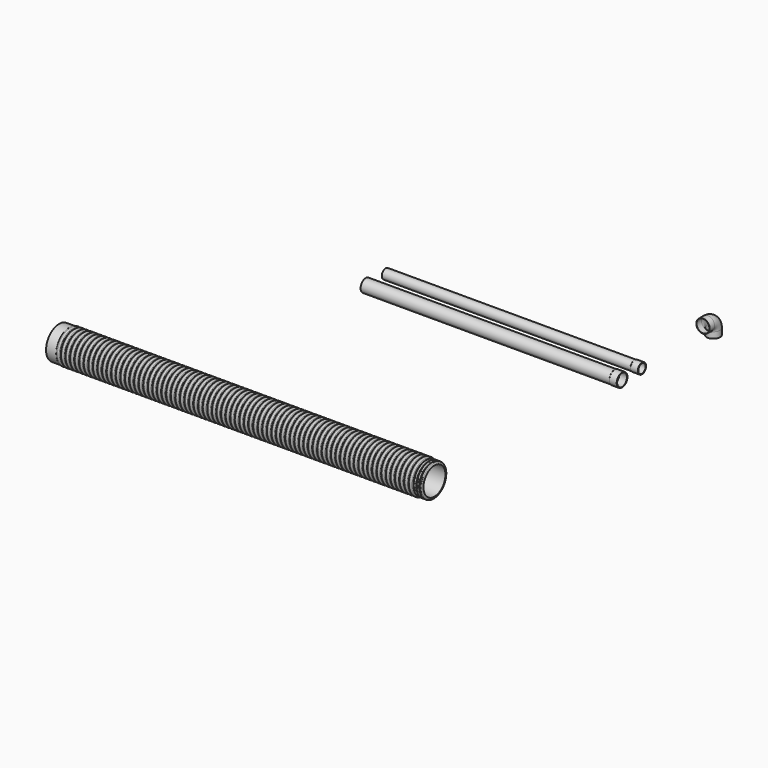
from build123d import *

# Parameters (mm, degrees)
F0_R      = 81.28
F0_R_2    = 76.2
F1_DEPTH  = 4140.2
F0_R_3    = 106.68
F0_R_4    = 101.6
F0_R_5    = 111.76
F2_DEPTH  = 127
F0_R_6    = 86.36
F3_DEPTH  = 127
F4_SIZE   = 5.07999
F4_2_SIZE = 5.07999
F9_R      = 111.76
F9_R_2    = 106.68


# Not quite as in the source:
# - a fillet or chamfer is up to 0.001 mm smaller than in the source, because OpenCascade refuses the exact size


with BuildPart() as f1:
    # F0 (on Right) → F1 (new body)
    with BuildSketch(Plane.YZ):
        with Locations((1112.0145320892, 0)):
            Circle(F0_R)
        with Locations((1112.0145320892, 0)):
            Circle(F0_R_2, mode=Mode.SUBTRACT)
    extrude(amount=-F1_DEPTH)

    # F0 (on Right) → F3 (join)
    with BuildSketch(Plane.YZ):
        with Locations((1112.0145320892, 0)):
            Circle(F0_R_6)
        with Locations((1112.0145320892, 0)):
            Circle(F0_R, mode=Mode.SUBTRACT)
        with Locations((1112.0145320892, 0)):
            Circle(F0_R)
        with Locations((1112.0145320892, 0)):
            Circle(F0_R_2, mode=Mode.SUBTRACT)
    extrude(amount=F3_DEPTH)

    # F4 (size 5.08 in the source; OpenCascade refuses exactly that, so slightly less here)
    f4_edges = [f1.edges().sort_by_distance(p)[0] for p in [
        (0, 1025.654532, 0),
    ]]
    chamfer(f4_edges, length=F4_SIZE)


with BuildPart() as f1b:
    # F0 (on Right) → F1, piece 2 (new body)
    with BuildSketch(Plane.YZ):
        with Locations((697.3502039909, 0)):
            Circle(F0_R_3)
        with Locations((697.3502039909, 0)):
            Circle(F0_R_4, mode=Mode.SUBTRACT)
    extrude(amount=-F1_DEPTH)

    # F0 (on Right) → F2 (join)
    with BuildSketch(Plane.YZ):
        with Locations((697.3502039909, 0)):
            Circle(F0_R_5)
        with Locations((697.3502039909, 0)):
            Circle(F0_R_3, mode=Mode.SUBTRACT)
        with Locations((697.3502039909, 0)):
            Circle(F0_R_3)
        with Locations((697.3502039909, 0)):
            Circle(F0_R_4, mode=Mode.SUBTRACT)
    extrude(amount=F2_DEPTH)

    # F4#2 (size 5.08 in the source; OpenCascade refuses exactly that, so slightly less here)
    f4_2_edges = [f1b.edges().sort_by_distance(p)[0] for p in [
        (0, 585.590204, 0),
    ]]
    chamfer(f4_2_edges, length=F4_2_SIZE)


with BuildPart() as f7:
    # F6 (on offset) → F7 (revolve)
    with BuildSketch(Plane.XZ.offset(3048)):
        with BuildLine():
            Line((-6096, 228.6), (0, 228.6))
            Line((0, 228.6), (0, 233.68))
            Line((0, 233.68), (-10.4299304682, 258.860079591))
            ThreePointArc((-10.4299304682, 258.860079591), (-15.1074585718, 264.5596640762), (-22.1632005311, 266.7))
            Line((-22.1632005311, 266.7), (-28.6367994689, 266.7))
            ThreePointArc((-28.6367994689, 266.7), (-35.6925414282, 264.5596640762), (-40.3700695318, 258.860079591))
            Line((-40.3700695318, 258.860079591), (-44.9333649686, 247.8433098584))
            ThreePointArc((-44.9333649686, 247.8433098584), (-50.8, 243.9233496539), (-56.6666350314, 247.8433098584))
            Line((-56.6666350314, 247.8433098584), (-61.2299304682, 258.860079591))
            ThreePointArc((-61.2299304682, 258.860079591), (-65.9074585718, 264.5596640762), (-72.9632005311, 266.7))
            Line((-72.9632005311, 266.7), (-79.4367994689, 266.7))
            ThreePointArc((-79.4367994689, 266.7), (-86.4925414282, 264.5596640762), (-91.1700695318, 258.860079591))
            Line((-91.1700695318, 258.860079591), (-95.7333649686, 247.8433098584))
            ThreePointArc((-95.7333649686, 247.8433098584), (-101.6, 243.9233496539), (-107.4666350314, 247.8433098584))
            Line((-107.4666350314, 247.8433098584), (-112.0299304682, 258.860079591))
            ThreePointArc((-112.0299304682, 258.860079591), (-116.7074585718, 264.5596640762), (-123.7632005311, 266.7))
            Line((-123.7632005311, 266.7), (-130.2367994689, 266.7))
            ThreePointArc((-130.2367994689, 266.7), (-137.2925414282, 264.5596640762), (-141.9700695318, 258.860079591))
            Line((-141.9700695318, 258.860079591), (-146.5333649686, 247.8433098584))
            ThreePointArc((-146.5333649686, 247.8433098584), (-152.4, 243.9233496539), (-158.2666350314, 247.8433098584))
            Line((-158.2666350314, 247.8433098584), (-166.4667420297, 267.6401193866))
            ThreePointArc((-166.4667420297, 267.6401193866), (-173.483034185, 276.1894961144), (-184.0666471241, 279.4))
            Line((-184.0666471241, 279.4), (-196.9333528759, 279.4))
            ThreePointArc((-196.9333528759, 279.4), (-207.516965815, 276.1894961144), (-214.5332579703, 267.6401193866))
            Line((-214.5332579703, 267.6401193866), (-219.8000474528, 254.9249647876))
            ThreePointArc((-219.8000474528, 254.9249647876), (-228.6, 249.0450244809), (-237.3999525472, 254.9249647876))
            Line((-237.3999525472, 254.9249647876), (-242.6667420297, 267.6401193866))
            ThreePointArc((-242.6667420297, 267.6401193866), (-249.683034185, 276.1894961144), (-260.2666471241, 279.4))
            Line((-260.2666471241, 279.4), (-273.1333528759, 279.4))
            ThreePointArc((-273.1333528759, 279.4), (-283.716965815, 276.1894961144), (-290.7332579703, 267.6401193866))
            Line((-290.7332579703, 267.6401193866), (-296.0000474528, 254.9249647876))
            ThreePointArc((-296.0000474528, 254.9249647876), (-304.8, 249.0450244809), (-313.5999525472, 254.9249647876))
            Line((-313.5999525472, 254.9249647876), (-318.8667420297, 267.6401193866))
            ThreePointArc((-318.8667420297, 267.6401193866), (-325.883034185, 276.1894961144), (-336.4666471241, 279.4))
            Line((-336.4666471241, 279.4), (-349.3333528759, 279.4))
            ThreePointArc((-349.3333528759, 279.4), (-359.916965815, 276.1894961144), (-366.9332579703, 267.6401193866))
            Line((-366.9332579703, 267.6401193866), (-372.2000474528, 254.9249647876))
            ThreePointArc((-372.2000474528, 254.9249647876), (-381, 249.0450244809), (-389.7999525472, 254.9249647876))
            Line((-389.7999525472, 254.9249647876), (-395.0667420297, 267.6401193866))
            ThreePointArc((-395.0667420297, 267.6401193866), (-402.083034185, 276.1894961144), (-412.6666471241, 279.4))
            Line((-412.6666471241, 279.4), (-425.5333528759, 279.4))
            ThreePointArc((-425.5333528759, 279.4), (-436.116965815, 276.1894961144), (-443.1332579703, 267.6401193866))
            Line((-443.1332579703, 267.6401193866), (-448.4000474528, 254.9249647876))
            ThreePointArc((-448.4000474528, 254.9249647876), (-457.2, 249.0450244809), (-465.9999525472, 254.9249647876))
            Line((-465.9999525472, 254.9249647876), (-471.2667420297, 267.6401193866))
            ThreePointArc((-471.2667420297, 267.6401193866), (-478.283034185, 276.1894961144), (-488.8666471241, 279.4))
            Line((-488.8666471241, 279.4), (-501.7333528759, 279.4))
            ThreePointArc((-501.7333528759, 279.4), (-512.316965815, 276.1894961144), (-519.3332579703, 267.6401193866))
            Line((-519.3332579703, 267.6401193866), (-524.6000474528, 254.9249647876))
            ThreePointArc((-524.6000474528, 254.9249647876), (-533.4, 249.0450244809), (-542.1999525472, 254.9249647876))
            Line((-542.1999525472, 254.9249647876), (-547.4667420297, 267.6401193866))
            ThreePointArc((-547.4667420297, 267.6401193866), (-554.483034185, 276.1894961144), (-565.0666471241, 279.4))
            Line((-565.0666471241, 279.4), (-577.9333528759, 279.4))
            ThreePointArc((-577.9333528759, 279.4), (-588.516965815, 276.1894961144), (-595.5332579703, 267.6401193866))
            Line((-595.5332579703, 267.6401193866), (-600.8000474528, 254.9249647876))
            ThreePointArc((-600.8000474528, 254.9249647876), (-609.6, 249.0450244809), (-618.3999525472, 254.9249647876))
            Line((-618.3999525472, 254.9249647876), (-623.6667420297, 267.6401193866))
            ThreePointArc((-623.6667420297, 267.6401193866), (-630.683034185, 276.1894961144), (-641.2666471241, 279.4))
            Line((-641.2666471241, 279.4), (-654.1333528759, 279.4))
            ThreePointArc((-654.1333528759, 279.4), (-664.716965815, 276.1894961144), (-671.7332579703, 267.6401193866))
            Line((-671.7332579703, 267.6401193866), (-677.0000474528, 254.9249647876))
            ThreePointArc((-677.0000474528, 254.9249647876), (-685.8, 249.0450244809), (-694.5999525472, 254.9249647876))
            Line((-694.5999525472, 254.9249647876), (-699.8667420297, 267.6401193866))
            ThreePointArc((-699.8667420297, 267.6401193866), (-706.883034185, 276.1894961144), (-717.4666471241, 279.4))
            Line((-717.4666471241, 279.4), (-730.3333528759, 279.4))
            ThreePointArc((-730.3333528759, 279.4), (-740.916965815, 276.1894961144), (-747.9332579703, 267.6401193866))
            Line((-747.9332579703, 267.6401193866), (-753.2000474528, 254.9249647876))
            ThreePointArc((-753.2000474528, 254.9249647876), (-762, 249.0450244809), (-770.7999525472, 254.9249647876))
            Line((-770.7999525472, 254.9249647876), (-776.0667420297, 267.6401193866))
            ThreePointArc((-776.0667420297, 267.6401193866), (-783.083034185, 276.1894961144), (-793.6666471241, 279.4))
            Line((-793.6666471241, 279.4), (-806.5333528759, 279.4))
            ThreePointArc((-806.5333528759, 279.4), (-817.116965815, 276.1894961144), (-824.1332579703, 267.6401193866))
            Line((-824.1332579703, 267.6401193866), (-829.4000474528, 254.9249647876))
            ThreePointArc((-829.4000474528, 254.9249647876), (-838.2, 249.0450244809), (-846.9999525472, 254.9249647876))
            Line((-846.9999525472, 254.9249647876), (-852.2667420297, 267.6401193866))
            ThreePointArc((-852.2667420297, 267.6401193866), (-859.283034185, 276.1894961144), (-869.8666471241, 279.4))
            Line((-869.8666471241, 279.4), (-882.7333528759, 279.4))
            ThreePointArc((-882.7333528759, 279.4), (-893.316965815, 276.1894961144), (-900.3332579703, 267.6401193866))
            Line((-900.3332579703, 267.6401193866), (-905.6000474528, 254.9249647876))
            ThreePointArc((-905.6000474528, 254.9249647876), (-914.4, 249.0450244809), (-923.1999525472, 254.9249647876))
            Line((-923.1999525472, 254.9249647876), (-928.4667420297, 267.6401193866))
            ThreePointArc((-928.4667420297, 267.6401193866), (-935.483034185, 276.1894961144), (-946.0666471241, 279.4))
            Line((-946.0666471241, 279.4), (-958.9333528759, 279.4))
            ThreePointArc((-958.9333528759, 279.4), (-969.516965815, 276.1894961144), (-976.5332579703, 267.6401193866))
            Line((-976.5332579703, 267.6401193866), (-981.8000474528, 254.9249647876))
            ThreePointArc((-981.8000474528, 254.9249647876), (-990.6, 249.0450244809), (-999.3999525472, 254.9249647876))
            Line((-999.3999525472, 254.9249647876), (-1004.6667420297, 267.6401193866))
            ThreePointArc((-1004.6667420297, 267.6401193866), (-1011.683034185, 276.1894961144), (-1022.2666471241, 279.4))
            Line((-1022.2666471241, 279.4), (-1035.1333528759, 279.4))
            ThreePointArc((-1035.1333528759, 279.4), (-1045.716965815, 276.1894961144), (-1052.7332579703, 267.6401193866))
            Line((-1052.7332579703, 267.6401193866), (-1058.0000474528, 254.9249647876))
            ThreePointArc((-1058.0000474528, 254.9249647876), (-1066.8, 249.0450244809), (-1075.5999525472, 254.9249647876))
            Line((-1075.5999525472, 254.9249647876), (-1080.8667420297, 267.6401193866))
            ThreePointArc((-1080.8667420297, 267.6401193866), (-1087.883034185, 276.1894961144), (-1098.4666471241, 279.4))
            Line((-1098.4666471241, 279.4), (-1111.3333528759, 279.4))
            ThreePointArc((-1111.3333528759, 279.4), (-1121.916965815, 276.1894961144), (-1128.9332579703, 267.6401193866))
            Line((-1128.9332579703, 267.6401193866), (-1134.2000474528, 254.9249647876))
            ThreePointArc((-1134.2000474528, 254.9249647876), (-1143, 249.0450244809), (-1151.7999525472, 254.9249647876))
            Line((-1151.7999525472, 254.9249647876), (-1157.0667420297, 267.6401193866))
            ThreePointArc((-1157.0667420297, 267.6401193866), (-1164.083034185, 276.1894961144), (-1174.6666471241, 279.4))
            Line((-1174.6666471241, 279.4), (-1187.5333528759, 279.4))
            ThreePointArc((-1187.5333528759, 279.4), (-1198.116965815, 276.1894961144), (-1205.1332579703, 267.6401193866))
            Line((-1205.1332579703, 267.6401193866), (-1210.4000474528, 254.9249647876))
            ThreePointArc((-1210.4000474528, 254.9249647876), (-1219.2, 249.0450244809), (-1227.9999525472, 254.9249647876))
            Line((-1227.9999525472, 254.9249647876), (-1233.2667420297, 267.6401193866))
            ThreePointArc((-1233.2667420297, 267.6401193866), (-1240.283034185, 276.1894961144), (-1250.8666471241, 279.4))
            Line((-1250.8666471241, 279.4), (-1263.7333528759, 279.4))
            ThreePointArc((-1263.7333528759, 279.4), (-1274.316965815, 276.1894961144), (-1281.3332579703, 267.6401193866))
            Line((-1281.3332579703, 267.6401193866), (-1286.6000474528, 254.9249647876))
            ThreePointArc((-1286.6000474528, 254.9249647876), (-1295.4, 249.0450244809), (-1304.1999525472, 254.9249647876))
            Line((-1304.1999525472, 254.9249647876), (-1309.4667420297, 267.6401193866))
            ThreePointArc((-1309.4667420297, 267.6401193866), (-1316.483034185, 276.1894961144), (-1327.0666471241, 279.4))
            Line((-1327.0666471241, 279.4), (-1339.9333528759, 279.4))
            ThreePointArc((-1339.9333528759, 279.4), (-1350.516965815, 276.1894961144), (-1357.5332579703, 267.6401193866))
            Line((-1357.5332579703, 267.6401193866), (-1362.8000474528, 254.9249647876))
            ThreePointArc((-1362.8000474528, 254.9249647876), (-1371.6, 249.0450244809), (-1380.3999525472, 254.9249647876))
            Line((-1380.3999525472, 254.9249647876), (-1385.6667420297, 267.6401193866))
            ThreePointArc((-1385.6667420297, 267.6401193866), (-1392.683034185, 276.1894961144), (-1403.2666471241, 279.4))
            Line((-1403.2666471241, 279.4), (-1416.1333528759, 279.4))
            ThreePointArc((-1416.1333528759, 279.4), (-1426.716965815, 276.1894961144), (-1433.7332579703, 267.6401193866))
            Line((-1433.7332579703, 267.6401193866), (-1439.0000474528, 254.9249647876))
            ThreePointArc((-1439.0000474528, 254.9249647876), (-1447.8, 249.0450244809), (-1456.5999525472, 254.9249647876))
            Line((-1456.5999525472, 254.9249647876), (-1461.8667420297, 267.6401193866))
            ThreePointArc((-1461.8667420297, 267.6401193866), (-1468.883034185, 276.1894961144), (-1479.4666471241, 279.4))
            Line((-1479.4666471241, 279.4), (-1492.3333528759, 279.4))
            ThreePointArc((-1492.3333528759, 279.4), (-1502.916965815, 276.1894961144), (-1509.9332579703, 267.6401193866))
            Line((-1509.9332579703, 267.6401193866), (-1515.2000474528, 254.9249647876))
            ThreePointArc((-1515.2000474528, 254.9249647876), (-1524, 249.0450244809), (-1532.7999525472, 254.9249647876))
            Line((-1532.7999525472, 254.9249647876), (-1538.0667420297, 267.6401193866))
            ThreePointArc((-1538.0667420297, 267.6401193866), (-1545.083034185, 276.1894961144), (-1555.6666471241, 279.4))
            Line((-1555.6666471241, 279.4), (-1568.5333528759, 279.4))
            ThreePointArc((-1568.5333528759, 279.4), (-1579.116965815, 276.1894961144), (-1586.1332579703, 267.6401193866))
            Line((-1586.1332579703, 267.6401193866), (-1591.4000474528, 254.9249647876))
            ThreePointArc((-1591.4000474528, 254.9249647876), (-1600.2, 249.0450244809), (-1608.9999525472, 254.9249647876))
            Line((-1608.9999525472, 254.9249647876), (-1614.2667420297, 267.6401193866))
            ThreePointArc((-1614.2667420297, 267.6401193866), (-1621.283034185, 276.1894961144), (-1631.8666471241, 279.4))
            Line((-1631.8666471241, 279.4), (-1644.7333528759, 279.4))
            ThreePointArc((-1644.7333528759, 279.4), (-1655.316965815, 276.1894961144), (-1662.3332579703, 267.6401193866))
            Line((-1662.3332579703, 267.6401193866), (-1667.6000474528, 254.9249647876))
            ThreePointArc((-1667.6000474528, 254.9249647876), (-1676.4, 249.0450244809), (-1685.1999525472, 254.9249647876))
            Line((-1685.1999525472, 254.9249647876), (-1690.4667420297, 267.6401193866))
            ThreePointArc((-1690.4667420297, 267.6401193866), (-1697.483034185, 276.1894961144), (-1708.0666471241, 279.4))
            Line((-1708.0666471241, 279.4), (-1720.9333528759, 279.4))
            ThreePointArc((-1720.9333528759, 279.4), (-1731.516965815, 276.1894961144), (-1738.5332579703, 267.6401193866))
            Line((-1738.5332579703, 267.6401193866), (-1743.8000474528, 254.9249647876))
            ThreePointArc((-1743.8000474528, 254.9249647876), (-1752.6, 249.0450244809), (-1761.3999525472, 254.9249647876))
            Line((-1761.3999525472, 254.9249647876), (-1766.6667420297, 267.6401193866))
            ThreePointArc((-1766.6667420297, 267.6401193866), (-1773.683034185, 276.1894961144), (-1784.2666471241, 279.4))
            Line((-1784.2666471241, 279.4), (-1797.1333528759, 279.4))
            ThreePointArc((-1797.1333528759, 279.4), (-1807.716965815, 276.1894961144), (-1814.7332579703, 267.6401193866))
            Line((-1814.7332579703, 267.6401193866), (-1820.0000474528, 254.9249647876))
            ThreePointArc((-1820.0000474528, 254.9249647876), (-1828.8, 249.0450244809), (-1837.5999525472, 254.9249647876))
            Line((-1837.5999525472, 254.9249647876), (-1842.8667420297, 267.6401193866))
            ThreePointArc((-1842.8667420297, 267.6401193866), (-1849.883034185, 276.1894961144), (-1860.4666471241, 279.4))
            Line((-1860.4666471241, 279.4), (-1873.3333528759, 279.4))
            ThreePointArc((-1873.3333528759, 279.4), (-1883.916965815, 276.1894961144), (-1890.9332579703, 267.6401193866))
            Line((-1890.9332579703, 267.6401193866), (-1896.2000474528, 254.9249647876))
            ThreePointArc((-1896.2000474528, 254.9249647876), (-1905, 249.0450244809), (-1913.7999525472, 254.9249647876))
            Line((-1913.7999525472, 254.9249647876), (-1919.0667420297, 267.6401193866))
            ThreePointArc((-1919.0667420297, 267.6401193866), (-1926.083034185, 276.1894961144), (-1936.6666471241, 279.4))
            Line((-1936.6666471241, 279.4), (-1949.5333528759, 279.4))
            ThreePointArc((-1949.5333528759, 279.4), (-1960.116965815, 276.1894961144), (-1967.1332579703, 267.6401193866))
            Line((-1967.1332579703, 267.6401193866), (-1972.4000474528, 254.9249647876))
            ThreePointArc((-1972.4000474528, 254.9249647876), (-1981.2, 249.0450244809), (-1989.9999525472, 254.9249647876))
            Line((-1989.9999525472, 254.9249647876), (-1995.2667420297, 267.6401193866))
            ThreePointArc((-1995.2667420297, 267.6401193866), (-2002.283034185, 276.1894961144), (-2012.8666471241, 279.4))
            Line((-2012.8666471241, 279.4), (-2025.7333528759, 279.4))
            ThreePointArc((-2025.7333528759, 279.4), (-2036.316965815, 276.1894961144), (-2043.3332579703, 267.6401193866))
            Line((-2043.3332579703, 267.6401193866), (-2048.6000474528, 254.9249647876))
            ThreePointArc((-2048.6000474528, 254.9249647876), (-2057.4, 249.0450244809), (-2066.1999525472, 254.9249647876))
            Line((-2066.1999525472, 254.9249647876), (-2071.4667420297, 267.6401193866))
            ThreePointArc((-2071.4667420297, 267.6401193866), (-2078.483034185, 276.1894961144), (-2089.0666471241, 279.4))
            Line((-2089.0666471241, 279.4), (-2101.9333528759, 279.4))
            ThreePointArc((-2101.9333528759, 279.4), (-2112.516965815, 276.1894961144), (-2119.5332579703, 267.6401193866))
            Line((-2119.5332579703, 267.6401193866), (-2124.8000474528, 254.9249647876))
            ThreePointArc((-2124.8000474528, 254.9249647876), (-2133.6, 249.0450244809), (-2142.3999525472, 254.9249647876))
            Line((-2142.3999525472, 254.9249647876), (-2147.6667420297, 267.6401193866))
            ThreePointArc((-2147.6667420297, 267.6401193866), (-2154.683034185, 276.1894961144), (-2165.2666471241, 279.4))
            Line((-2165.2666471241, 279.4), (-2178.1333528759, 279.4))
            ThreePointArc((-2178.1333528759, 279.4), (-2188.716965815, 276.1894961144), (-2195.7332579703, 267.6401193866))
            Line((-2195.7332579703, 267.6401193866), (-2201.0000474528, 254.9249647876))
            ThreePointArc((-2201.0000474528, 254.9249647876), (-2209.8, 249.0450244809), (-2218.5999525472, 254.9249647876))
            Line((-2218.5999525472, 254.9249647876), (-2223.8667420297, 267.6401193866))
            ThreePointArc((-2223.8667420297, 267.6401193866), (-2230.883034185, 276.1894961144), (-2241.4666471241, 279.4))
            Line((-2241.4666471241, 279.4), (-2254.3333528759, 279.4))
            ThreePointArc((-2254.3333528759, 279.4), (-2264.916965815, 276.1894961144), (-2271.9332579703, 267.6401193866))
            Line((-2271.9332579703, 267.6401193866), (-2277.2000474528, 254.9249647876))
            ThreePointArc((-2277.2000474528, 254.9249647876), (-2286, 249.0450244809), (-2294.7999525472, 254.9249647876))
            Line((-2294.7999525472, 254.9249647876), (-2300.0667420297, 267.6401193866))
            ThreePointArc((-2300.0667420297, 267.6401193866), (-2307.083034185, 276.1894961144), (-2317.6666471241, 279.4))
            Line((-2317.6666471241, 279.4), (-2330.5333528759, 279.4))
            ThreePointArc((-2330.5333528759, 279.4), (-2341.116965815, 276.1894961144), (-2348.1332579703, 267.6401193866))
            Line((-2348.1332579703, 267.6401193866), (-2353.4000474528, 254.9249647876))
            ThreePointArc((-2353.4000474528, 254.9249647876), (-2362.2, 249.0450244809), (-2370.9999525472, 254.9249647876))
            Line((-2370.9999525472, 254.9249647876), (-2376.2667420297, 267.6401193866))
            ThreePointArc((-2376.2667420297, 267.6401193866), (-2383.283034185, 276.1894961144), (-2393.8666471241, 279.4))
            Line((-2393.8666471241, 279.4), (-2406.7333528759, 279.4))
            ThreePointArc((-2406.7333528759, 279.4), (-2417.316965815, 276.1894961144), (-2424.3332579703, 267.6401193866))
            Line((-2424.3332579703, 267.6401193866), (-2429.6000474528, 254.9249647876))
            ThreePointArc((-2429.6000474528, 254.9249647876), (-2438.4, 249.0450244809), (-2447.1999525472, 254.9249647876))
            Line((-2447.1999525472, 254.9249647876), (-2452.4667420297, 267.6401193866))
            ThreePointArc((-2452.4667420297, 267.6401193866), (-2459.483034185, 276.1894961144), (-2470.0666471241, 279.4))
            Line((-2470.0666471241, 279.4), (-2482.9333528759, 279.4))
            ThreePointArc((-2482.9333528759, 279.4), (-2493.516965815, 276.1894961144), (-2500.5332579703, 267.6401193866))
            Line((-2500.5332579703, 267.6401193866), (-2505.8000474528, 254.9249647876))
            ThreePointArc((-2505.8000474528, 254.9249647876), (-2514.6, 249.0450244809), (-2523.3999525472, 254.9249647876))
            Line((-2523.3999525472, 254.9249647876), (-2528.6667420297, 267.6401193866))
            ThreePointArc((-2528.6667420297, 267.6401193866), (-2535.683034185, 276.1894961144), (-2546.2666471241, 279.4))
            Line((-2546.2666471241, 279.4), (-2559.1333528759, 279.4))
            ThreePointArc((-2559.1333528759, 279.4), (-2569.716965815, 276.1894961144), (-2576.7332579703, 267.6401193866))
            Line((-2576.7332579703, 267.6401193866), (-2582.0000474528, 254.9249647876))
            ThreePointArc((-2582.0000474528, 254.9249647876), (-2590.8, 249.0450244809), (-2599.5999525472, 254.9249647876))
            Line((-2599.5999525472, 254.9249647876), (-2604.8667420297, 267.6401193866))
            ThreePointArc((-2604.8667420297, 267.6401193866), (-2611.883034185, 276.1894961144), (-2622.4666471241, 279.4))
            Line((-2622.4666471241, 279.4), (-2635.3333528759, 279.4))
            ThreePointArc((-2635.3333528759, 279.4), (-2645.916965815, 276.1894961144), (-2652.9332579703, 267.6401193866))
            Line((-2652.9332579703, 267.6401193866), (-2658.2000474528, 254.9249647876))
            ThreePointArc((-2658.2000474528, 254.9249647876), (-2667, 249.0450244809), (-2675.7999525472, 254.9249647876))
            Line((-2675.7999525472, 254.9249647876), (-2681.0667420297, 267.6401193866))
            ThreePointArc((-2681.0667420297, 267.6401193866), (-2688.083034185, 276.1894961144), (-2698.6666471241, 279.4))
            Line((-2698.6666471241, 279.4), (-2711.5333528759, 279.4))
            ThreePointArc((-2711.5333528759, 279.4), (-2722.116965815, 276.1894961144), (-2729.1332579703, 267.6401193866))
            Line((-2729.1332579703, 267.6401193866), (-2734.4000474528, 254.9249647876))
            ThreePointArc((-2734.4000474528, 254.9249647876), (-2743.2, 249.0450244809), (-2751.9999525472, 254.9249647876))
            Line((-2751.9999525472, 254.9249647876), (-2757.2667420297, 267.6401193866))
            ThreePointArc((-2757.2667420297, 267.6401193866), (-2764.283034185, 276.1894961144), (-2774.8666471241, 279.4))
            Line((-2774.8666471241, 279.4), (-2787.7333528759, 279.4))
            ThreePointArc((-2787.7333528759, 279.4), (-2798.316965815, 276.1894961144), (-2805.3332579703, 267.6401193866))
            Line((-2805.3332579703, 267.6401193866), (-2810.6000474528, 254.9249647876))
            ThreePointArc((-2810.6000474528, 254.9249647876), (-2819.4, 249.0450244809), (-2828.1999525472, 254.9249647876))
            Line((-2828.1999525472, 254.9249647876), (-2833.4667420297, 267.6401193866))
            ThreePointArc((-2833.4667420297, 267.6401193866), (-2840.483034185, 276.1894961144), (-2851.0666471241, 279.4))
            Line((-2851.0666471241, 279.4), (-2863.9333528759, 279.4))
            ThreePointArc((-2863.9333528759, 279.4), (-2874.516965815, 276.1894961144), (-2881.5332579703, 267.6401193866))
            Line((-2881.5332579703, 267.6401193866), (-2886.8000474528, 254.9249647876))
            ThreePointArc((-2886.8000474528, 254.9249647876), (-2895.6, 249.0450244809), (-2904.3999525472, 254.9249647876))
            Line((-2904.3999525472, 254.9249647876), (-2909.6667420297, 267.6401193866))
            ThreePointArc((-2909.6667420297, 267.6401193866), (-2916.683034185, 276.1894961144), (-2927.2666471241, 279.4))
            Line((-2927.2666471241, 279.4), (-2940.1333528759, 279.4))
            ThreePointArc((-2940.1333528759, 279.4), (-2950.716965815, 276.1894961144), (-2957.7332579703, 267.6401193866))
            Line((-2957.7332579703, 267.6401193866), (-2963.0000474528, 254.9249647876))
            ThreePointArc((-2963.0000474528, 254.9249647876), (-2971.8, 249.0450244809), (-2980.5999525472, 254.9249647876))
            Line((-2980.5999525472, 254.9249647876), (-2985.8667420297, 267.6401193866))
            ThreePointArc((-2985.8667420297, 267.6401193866), (-2992.883034185, 276.1894961144), (-3003.4666471241, 279.4))
            Line((-3003.4666471241, 279.4), (-3016.3333528759, 279.4))
            ThreePointArc((-3016.3333528759, 279.4), (-3026.916965815, 276.1894961144), (-3033.9332579703, 267.6401193866))
            Line((-3033.9332579703, 267.6401193866), (-3039.2000474528, 254.9249647876))
            ThreePointArc((-3039.2000474528, 254.9249647876), (-3048, 249.0450244809), (-3056.7999525472, 254.9249647876))
            Line((-3056.7999525472, 254.9249647876), (-3062.0667420297, 267.6401193866))
            ThreePointArc((-3062.0667420297, 267.6401193866), (-3069.083034185, 276.1894961144), (-3079.6666471241, 279.4))
            Line((-3079.6666471241, 279.4), (-3092.5333528759, 279.4))
            ThreePointArc((-3092.5333528759, 279.4), (-3103.116965815, 276.1894961144), (-3110.1332579703, 267.6401193866))
            Line((-3110.1332579703, 267.6401193866), (-3115.4000474528, 254.9249647876))
            ThreePointArc((-3115.4000474528, 254.9249647876), (-3124.2, 249.0450244809), (-3132.9999525472, 254.9249647876))
            Line((-3132.9999525472, 254.9249647876), (-3138.2667420297, 267.6401193866))
            ThreePointArc((-3138.2667420297, 267.6401193866), (-3145.283034185, 276.1894961144), (-3155.8666471241, 279.4))
            Line((-3155.8666471241, 279.4), (-3168.7333528759, 279.4))
            ThreePointArc((-3168.7333528759, 279.4), (-3179.316965815, 276.1894961144), (-3186.3332579703, 267.6401193866))
            Line((-3186.3332579703, 267.6401193866), (-3191.6000474528, 254.9249647876))
            ThreePointArc((-3191.6000474528, 254.9249647876), (-3200.4, 249.0450244809), (-3209.1999525472, 254.9249647876))
            Line((-3209.1999525472, 254.9249647876), (-3214.4667420297, 267.6401193866))
            ThreePointArc((-3214.4667420297, 267.6401193866), (-3221.483034185, 276.1894961144), (-3232.0666471241, 279.4))
            Line((-3232.0666471241, 279.4), (-3244.9333528759, 279.4))
            ThreePointArc((-3244.9333528759, 279.4), (-3255.516965815, 276.1894961144), (-3262.5332579703, 267.6401193866))
            Line((-3262.5332579703, 267.6401193866), (-3267.8000474528, 254.9249647876))
            ThreePointArc((-3267.8000474528, 254.9249647876), (-3276.6, 249.0450244809), (-3285.3999525472, 254.9249647876))
            Line((-3285.3999525472, 254.9249647876), (-3290.6667420297, 267.6401193866))
            ThreePointArc((-3290.6667420297, 267.6401193866), (-3297.683034185, 276.1894961144), (-3308.2666471241, 279.4))
            Line((-3308.2666471241, 279.4), (-3321.1333528759, 279.4))
            ThreePointArc((-3321.1333528759, 279.4), (-3331.716965815, 276.1894961144), (-3338.7332579703, 267.6401193866))
            Line((-3338.7332579703, 267.6401193866), (-3344.0000474528, 254.9249647876))
            ThreePointArc((-3344.0000474528, 254.9249647876), (-3352.8, 249.0450244809), (-3361.5999525472, 254.9249647876))
            Line((-3361.5999525472, 254.9249647876), (-3366.8667420297, 267.6401193866))
            ThreePointArc((-3366.8667420297, 267.6401193866), (-3373.883034185, 276.1894961144), (-3384.4666471241, 279.4))
            Line((-3384.4666471241, 279.4), (-3397.3333528759, 279.4))
            ThreePointArc((-3397.3333528759, 279.4), (-3407.916965815, 276.1894961144), (-3414.9332579703, 267.6401193866))
            Line((-3414.9332579703, 267.6401193866), (-3420.2000474528, 254.9249647876))
            ThreePointArc((-3420.2000474528, 254.9249647876), (-3429, 249.0450244809), (-3437.7999525472, 254.9249647876))
            Line((-3437.7999525472, 254.9249647876), (-3443.0667420297, 267.6401193866))
            ThreePointArc((-3443.0667420297, 267.6401193866), (-3450.083034185, 276.1894961144), (-3460.6666471241, 279.4))
            Line((-3460.6666471241, 279.4), (-3473.5333528759, 279.4))
            ThreePointArc((-3473.5333528759, 279.4), (-3484.116965815, 276.1894961144), (-3491.1332579703, 267.6401193866))
            Line((-3491.1332579703, 267.6401193866), (-3496.4000474528, 254.9249647876))
            ThreePointArc((-3496.4000474528, 254.9249647876), (-3505.2, 249.0450244809), (-3513.9999525472, 254.9249647876))
            Line((-3513.9999525472, 254.9249647876), (-3519.2667420297, 267.6401193866))
            ThreePointArc((-3519.2667420297, 267.6401193866), (-3526.283034185, 276.1894961144), (-3536.8666471241, 279.4))
            Line((-3536.8666471241, 279.4), (-3549.7333528759, 279.4))
            ThreePointArc((-3549.7333528759, 279.4), (-3560.316965815, 276.1894961144), (-3567.3332579703, 267.6401193866))
            Line((-3567.3332579703, 267.6401193866), (-3572.6000474528, 254.9249647876))
            ThreePointArc((-3572.6000474528, 254.9249647876), (-3581.4, 249.0450244809), (-3590.1999525472, 254.9249647876))
            Line((-3590.1999525472, 254.9249647876), (-3595.4667420297, 267.6401193866))
            ThreePointArc((-3595.4667420297, 267.6401193866), (-3602.483034185, 276.1894961144), (-3613.0666471241, 279.4))
            Line((-3613.0666471241, 279.4), (-3625.9333528759, 279.4))
            ThreePointArc((-3625.9333528759, 279.4), (-3636.516965815, 276.1894961144), (-3643.5332579703, 267.6401193866))
            Line((-3643.5332579703, 267.6401193866), (-3648.8000474528, 254.9249647876))
            ThreePointArc((-3648.8000474528, 254.9249647876), (-3657.6, 249.0450244809), (-3666.3999525472, 254.9249647876))
            Line((-3666.3999525472, 254.9249647876), (-3671.6667420297, 267.6401193866))
            ThreePointArc((-3671.6667420297, 267.6401193866), (-3678.683034185, 276.1894961144), (-3689.2666471241, 279.4))
            Line((-3689.2666471241, 279.4), (-3702.1333528759, 279.4))
            ThreePointArc((-3702.1333528759, 279.4), (-3712.716965815, 276.1894961144), (-3719.7332579703, 267.6401193866))
            Line((-3719.7332579703, 267.6401193866), (-3725.0000474528, 254.9249647876))
            ThreePointArc((-3725.0000474528, 254.9249647876), (-3733.8, 249.0450244809), (-3742.5999525472, 254.9249647876))
            Line((-3742.5999525472, 254.9249647876), (-3747.8667420297, 267.6401193866))
            ThreePointArc((-3747.8667420297, 267.6401193866), (-3754.883034185, 276.1894961144), (-3765.4666471241, 279.4))
            Line((-3765.4666471241, 279.4), (-3778.3333528759, 279.4))
            ThreePointArc((-3778.3333528759, 279.4), (-3788.916965815, 276.1894961144), (-3795.9332579703, 267.6401193866))
            Line((-3795.9332579703, 267.6401193866), (-3801.2000474528, 254.9249647876))
            ThreePointArc((-3801.2000474528, 254.9249647876), (-3810, 249.0450244809), (-3818.7999525472, 254.9249647876))
            Line((-3818.7999525472, 254.9249647876), (-3824.0667420297, 267.6401193866))
            ThreePointArc((-3824.0667420297, 267.6401193866), (-3831.083034185, 276.1894961144), (-3841.6666471241, 279.4))
            Line((-3841.6666471241, 279.4), (-3854.5333528759, 279.4))
            ThreePointArc((-3854.5333528759, 279.4), (-3865.116965815, 276.1894961144), (-3872.1332579703, 267.6401193866))
            Line((-3872.1332579703, 267.6401193866), (-3877.4000474528, 254.9249647876))
            ThreePointArc((-3877.4000474528, 254.9249647876), (-3886.2, 249.0450244809), (-3894.9999525472, 254.9249647876))
            Line((-3894.9999525472, 254.9249647876), (-3900.2667420297, 267.6401193866))
            ThreePointArc((-3900.2667420297, 267.6401193866), (-3907.283034185, 276.1894961144), (-3917.8666471241, 279.4))
            Line((-3917.8666471241, 279.4), (-3930.7333528759, 279.4))
            ThreePointArc((-3930.7333528759, 279.4), (-3941.316965815, 276.1894961144), (-3948.3332579703, 267.6401193866))
            Line((-3948.3332579703, 267.6401193866), (-3953.6000474528, 254.9249647876))
            ThreePointArc((-3953.6000474528, 254.9249647876), (-3962.4, 249.0450244809), (-3971.1999525472, 254.9249647876))
            Line((-3971.1999525472, 254.9249647876), (-3976.4667420297, 267.6401193866))
            ThreePointArc((-3976.4667420297, 267.6401193866), (-3983.483034185, 276.1894961144), (-3994.0666471241, 279.4))
            Line((-3994.0666471241, 279.4), (-4006.9333528759, 279.4))
            ThreePointArc((-4006.9333528759, 279.4), (-4017.516965815, 276.1894961144), (-4024.5332579703, 267.6401193866))
            Line((-4024.5332579703, 267.6401193866), (-4029.8000474528, 254.9249647876))
            ThreePointArc((-4029.8000474528, 254.9249647876), (-4038.6, 249.0450244809), (-4047.3999525472, 254.9249647876))
            Line((-4047.3999525472, 254.9249647876), (-4052.6667420297, 267.6401193866))
            ThreePointArc((-4052.6667420297, 267.6401193866), (-4059.683034185, 276.1894961144), (-4070.2666471241, 279.4))
            Line((-4070.2666471241, 279.4), (-4083.1333528759, 279.4))
            ThreePointArc((-4083.1333528759, 279.4), (-4093.716965815, 276.1894961144), (-4100.7332579703, 267.6401193866))
            Line((-4100.7332579703, 267.6401193866), (-4106.0000474528, 254.9249647876))
            ThreePointArc((-4106.0000474528, 254.9249647876), (-4114.8, 249.0450244809), (-4123.5999525472, 254.9249647876))
            Line((-4123.5999525472, 254.9249647876), (-4128.8667420297, 267.6401193866))
            ThreePointArc((-4128.8667420297, 267.6401193866), (-4135.883034185, 276.1894961144), (-4146.4666471241, 279.4))
            Line((-4146.4666471241, 279.4), (-4159.3333528759, 279.4))
            ThreePointArc((-4159.3333528759, 279.4), (-4169.916965815, 276.1894961144), (-4176.9332579703, 267.6401193866))
            Line((-4176.9332579703, 267.6401193866), (-4182.2000474528, 254.9249647876))
            ThreePointArc((-4182.2000474528, 254.9249647876), (-4191, 249.0450244809), (-4199.7999525472, 254.9249647876))
            Line((-4199.7999525472, 254.9249647876), (-4205.0667420297, 267.6401193866))
            ThreePointArc((-4205.0667420297, 267.6401193866), (-4212.083034185, 276.1894961144), (-4222.6666471241, 279.4))
            Line((-4222.6666471241, 279.4), (-4235.5333528759, 279.4))
            ThreePointArc((-4235.5333528759, 279.4), (-4246.116965815, 276.1894961144), (-4253.1332579703, 267.6401193866))
            Line((-4253.1332579703, 267.6401193866), (-4258.4000474528, 254.9249647876))
            ThreePointArc((-4258.4000474528, 254.9249647876), (-4267.2, 249.0450244809), (-4275.9999525472, 254.9249647876))
            Line((-4275.9999525472, 254.9249647876), (-4281.2667420297, 267.6401193866))
            ThreePointArc((-4281.2667420297, 267.6401193866), (-4288.283034185, 276.1894961144), (-4298.8666471241, 279.4))
            Line((-4298.8666471241, 279.4), (-4311.7333528759, 279.4))
            ThreePointArc((-4311.7333528759, 279.4), (-4322.316965815, 276.1894961144), (-4329.3332579703, 267.6401193866))
            Line((-4329.3332579703, 267.6401193866), (-4334.6000474528, 254.9249647876))
            ThreePointArc((-4334.6000474528, 254.9249647876), (-4343.4, 249.0450244809), (-4352.1999525472, 254.9249647876))
            Line((-4352.1999525472, 254.9249647876), (-4357.4667420297, 267.6401193866))
            ThreePointArc((-4357.4667420297, 267.6401193866), (-4364.483034185, 276.1894961144), (-4375.0666471241, 279.4))
            Line((-4375.0666471241, 279.4), (-4387.9333528759, 279.4))
            ThreePointArc((-4387.9333528759, 279.4), (-4398.516965815, 276.1894961144), (-4405.5332579703, 267.6401193866))
            Line((-4405.5332579703, 267.6401193866), (-4410.8000474528, 254.9249647876))
            ThreePointArc((-4410.8000474528, 254.9249647876), (-4419.6, 249.0450244809), (-4428.3999525472, 254.9249647876))
            Line((-4428.3999525472, 254.9249647876), (-4433.6667420297, 267.6401193866))
            ThreePointArc((-4433.6667420297, 267.6401193866), (-4440.683034185, 276.1894961144), (-4451.2666471241, 279.4))
            Line((-4451.2666471241, 279.4), (-4464.1333528759, 279.4))
            ThreePointArc((-4464.1333528759, 279.4), (-4474.716965815, 276.1894961144), (-4481.7332579703, 267.6401193866))
            Line((-4481.7332579703, 267.6401193866), (-4487.0000474528, 254.9249647876))
            ThreePointArc((-4487.0000474528, 254.9249647876), (-4495.8, 249.0450244809), (-4504.5999525472, 254.9249647876))
            Line((-4504.5999525472, 254.9249647876), (-4509.8667420297, 267.6401193866))
            ThreePointArc((-4509.8667420297, 267.6401193866), (-4516.883034185, 276.1894961144), (-4527.4666471241, 279.4))
            Line((-4527.4666471241, 279.4), (-4540.3333528759, 279.4))
            ThreePointArc((-4540.3333528759, 279.4), (-4550.916965815, 276.1894961144), (-4557.9332579703, 267.6401193866))
            Line((-4557.9332579703, 267.6401193866), (-4563.2000474528, 254.9249647876))
            ThreePointArc((-4563.2000474528, 254.9249647876), (-4572, 249.0450244809), (-4580.7999525472, 254.9249647876))
            Line((-4580.7999525472, 254.9249647876), (-4586.0667420297, 267.6401193866))
            ThreePointArc((-4586.0667420297, 267.6401193866), (-4593.083034185, 276.1894961144), (-4603.6666471241, 279.4))
            Line((-4603.6666471241, 279.4), (-4616.5333528759, 279.4))
            ThreePointArc((-4616.5333528759, 279.4), (-4627.116965815, 276.1894961144), (-4634.1332579703, 267.6401193866))
            Line((-4634.1332579703, 267.6401193866), (-4639.4000474528, 254.9249647876))
            ThreePointArc((-4639.4000474528, 254.9249647876), (-4648.2, 249.0450244809), (-4656.9999525472, 254.9249647876))
            Line((-4656.9999525472, 254.9249647876), (-4662.2667420297, 267.6401193866))
            ThreePointArc((-4662.2667420297, 267.6401193866), (-4669.283034185, 276.1894961144), (-4679.8666471241, 279.4))
            Line((-4679.8666471241, 279.4), (-4692.7333528759, 279.4))
            ThreePointArc((-4692.7333528759, 279.4), (-4703.316965815, 276.1894961144), (-4710.3332579703, 267.6401193866))
            Line((-4710.3332579703, 267.6401193866), (-4715.6000474528, 254.9249647876))
            ThreePointArc((-4715.6000474528, 254.9249647876), (-4724.4, 249.0450244809), (-4733.1999525472, 254.9249647876))
            Line((-4733.1999525472, 254.9249647876), (-4738.4667420297, 267.6401193866))
            ThreePointArc((-4738.4667420297, 267.6401193866), (-4745.483034185, 276.1894961144), (-4756.0666471241, 279.4))
            Line((-4756.0666471241, 279.4), (-4768.9333528759, 279.4))
            ThreePointArc((-4768.9333528759, 279.4), (-4779.516965815, 276.1894961144), (-4786.5332579703, 267.6401193866))
            Line((-4786.5332579703, 267.6401193866), (-4791.8000474528, 254.9249647876))
            ThreePointArc((-4791.8000474528, 254.9249647876), (-4800.6, 249.0450244809), (-4809.3999525472, 254.9249647876))
            Line((-4809.3999525472, 254.9249647876), (-4814.6667420297, 267.6401193866))
            ThreePointArc((-4814.6667420297, 267.6401193866), (-4821.683034185, 276.1894961144), (-4832.2666471241, 279.4))
            Line((-4832.2666471241, 279.4), (-4845.1333528759, 279.4))
            ThreePointArc((-4845.1333528759, 279.4), (-4855.716965815, 276.1894961144), (-4862.7332579703, 267.6401193866))
            Line((-4862.7332579703, 267.6401193866), (-4868.0000474528, 254.9249647876))
            ThreePointArc((-4868.0000474528, 254.9249647876), (-4876.8, 249.0450244809), (-4885.5999525472, 254.9249647876))
            Line((-4885.5999525472, 254.9249647876), (-4890.8667420297, 267.6401193866))
            ThreePointArc((-4890.8667420297, 267.6401193866), (-4897.883034185, 276.1894961144), (-4908.4666471241, 279.4))
            Line((-4908.4666471241, 279.4), (-4921.3333528759, 279.4))
            ThreePointArc((-4921.3333528759, 279.4), (-4931.916965815, 276.1894961144), (-4938.9332579703, 267.6401193866))
            Line((-4938.9332579703, 267.6401193866), (-4944.2000474528, 254.9249647876))
            ThreePointArc((-4944.2000474528, 254.9249647876), (-4953, 249.0450244809), (-4961.7999525472, 254.9249647876))
            Line((-4961.7999525472, 254.9249647876), (-4967.0667420297, 267.6401193866))
            ThreePointArc((-4967.0667420297, 267.6401193866), (-4974.083034185, 276.1894961144), (-4984.6666471241, 279.4))
            Line((-4984.6666471241, 279.4), (-4997.5333528759, 279.4))
            ThreePointArc((-4997.5333528759, 279.4), (-5008.116965815, 276.1894961144), (-5015.1332579703, 267.6401193866))
            Line((-5015.1332579703, 267.6401193866), (-5020.4000474528, 254.9249647876))
            ThreePointArc((-5020.4000474528, 254.9249647876), (-5029.2, 249.0450244809), (-5037.9999525472, 254.9249647876))
            Line((-5037.9999525472, 254.9249647876), (-5043.2667420297, 267.6401193866))
            ThreePointArc((-5043.2667420297, 267.6401193866), (-5050.283034185, 276.1894961144), (-5060.8666471241, 279.4))
            Line((-5060.8666471241, 279.4), (-5073.7333528759, 279.4))
            ThreePointArc((-5073.7333528759, 279.4), (-5084.316965815, 276.1894961144), (-5091.3332579703, 267.6401193866))
            Line((-5091.3332579703, 267.6401193866), (-5096.6000474528, 254.9249647876))
            ThreePointArc((-5096.6000474528, 254.9249647876), (-5105.4, 249.0450244809), (-5114.1999525472, 254.9249647876))
            Line((-5114.1999525472, 254.9249647876), (-5119.4667420297, 267.6401193866))
            ThreePointArc((-5119.4667420297, 267.6401193866), (-5126.483034185, 276.1894961144), (-5137.0666471241, 279.4))
            Line((-5137.0666471241, 279.4), (-5149.9333528759, 279.4))
            ThreePointArc((-5149.9333528759, 279.4), (-5160.516965815, 276.1894961144), (-5167.5332579703, 267.6401193866))
            Line((-5167.5332579703, 267.6401193866), (-5172.8000474528, 254.9249647876))
            ThreePointArc((-5172.8000474528, 254.9249647876), (-5181.6, 249.0450244809), (-5190.3999525472, 254.9249647876))
            Line((-5190.3999525472, 254.9249647876), (-5195.6667420297, 267.6401193866))
            ThreePointArc((-5195.6667420297, 267.6401193866), (-5202.683034185, 276.1894961144), (-5213.2666471241, 279.4))
            Line((-5213.2666471241, 279.4), (-5226.1333528759, 279.4))
            ThreePointArc((-5226.1333528759, 279.4), (-5236.716965815, 276.1894961144), (-5243.7332579703, 267.6401193866))
            Line((-5243.7332579703, 267.6401193866), (-5249.0000474528, 254.9249647876))
            ThreePointArc((-5249.0000474528, 254.9249647876), (-5257.8, 249.0450244809), (-5266.5999525472, 254.9249647876))
            Line((-5266.5999525472, 254.9249647876), (-5271.8667420297, 267.6401193866))
            ThreePointArc((-5271.8667420297, 267.6401193866), (-5278.883034185, 276.1894961144), (-5289.4666471241, 279.4))
            Line((-5289.4666471241, 279.4), (-5302.3333528759, 279.4))
            ThreePointArc((-5302.3333528759, 279.4), (-5312.916965815, 276.1894961144), (-5319.9332579703, 267.6401193866))
            Line((-5319.9332579703, 267.6401193866), (-5325.2000474528, 254.9249647876))
            ThreePointArc((-5325.2000474528, 254.9249647876), (-5334, 249.0450244809), (-5342.7999525472, 254.9249647876))
            Line((-5342.7999525472, 254.9249647876), (-5348.0667420297, 267.6401193866))
            ThreePointArc((-5348.0667420297, 267.6401193866), (-5355.083034185, 276.1894961144), (-5365.6666471241, 279.4))
            Line((-5365.6666471241, 279.4), (-5378.5333528759, 279.4))
            ThreePointArc((-5378.5333528759, 279.4), (-5389.116965815, 276.1894961144), (-5396.1332579703, 267.6401193866))
            Line((-5396.1332579703, 267.6401193866), (-5401.4000474528, 254.9249647876))
            ThreePointArc((-5401.4000474528, 254.9249647876), (-5410.2, 249.0450244809), (-5418.9999525472, 254.9249647876))
            Line((-5418.9999525472, 254.9249647876), (-5424.2667420297, 267.6401193866))
            ThreePointArc((-5424.2667420297, 267.6401193866), (-5431.283034185, 276.1894961144), (-5441.8666471241, 279.4))
            Line((-5441.8666471241, 279.4), (-5454.7333528759, 279.4))
            ThreePointArc((-5454.7333528759, 279.4), (-5465.316965815, 276.1894961144), (-5472.3332579703, 267.6401193866))
            Line((-5472.3332579703, 267.6401193866), (-5477.6000474528, 254.9249647876))
            ThreePointArc((-5477.6000474528, 254.9249647876), (-5486.4, 249.0450244809), (-5495.1999525472, 254.9249647876))
            Line((-5495.1999525472, 254.9249647876), (-5500.4667420297, 267.6401193866))
            ThreePointArc((-5500.4667420297, 267.6401193866), (-5507.483034185, 276.1894961144), (-5518.0666471241, 279.4))
            Line((-5518.0666471241, 279.4), (-5530.9333528759, 279.4))
            ThreePointArc((-5530.9333528759, 279.4), (-5541.516965815, 276.1894961144), (-5548.5332579703, 267.6401193866))
            Line((-5548.5332579703, 267.6401193866), (-5553.8000474528, 254.9249647876))
            ThreePointArc((-5553.8000474528, 254.9249647876), (-5562.6, 249.0450244809), (-5571.3999525472, 254.9249647876))
            Line((-5571.3999525472, 254.9249647876), (-5576.6667420297, 267.6401193866))
            ThreePointArc((-5576.6667420297, 267.6401193866), (-5583.683034185, 276.1894961144), (-5594.2666471241, 279.4))
            Line((-5594.2666471241, 279.4), (-5607.1333528759, 279.4))
            ThreePointArc((-5607.1333528759, 279.4), (-5617.716965815, 276.1894961144), (-5624.7332579703, 267.6401193866))
            Line((-5624.7332579703, 267.6401193866), (-5630.0000474528, 254.9249647876))
            ThreePointArc((-5630.0000474528, 254.9249647876), (-5638.8, 249.0450244809), (-5647.5999525472, 254.9249647876))
            Line((-5647.5999525472, 254.9249647876), (-5652.8667420297, 267.6401193866))
            ThreePointArc((-5652.8667420297, 267.6401193866), (-5659.883034185, 276.1894961144), (-5670.4666471241, 279.4))
            Line((-5670.4666471241, 279.4), (-5683.3333528759, 279.4))
            ThreePointArc((-5683.3333528759, 279.4), (-5693.916965815, 276.1894961144), (-5700.9332579703, 267.6401193866))
            Line((-5700.9332579703, 267.6401193866), (-5706.2000474528, 254.9249647876))
            ThreePointArc((-5706.2000474528, 254.9249647876), (-5715, 249.0450244809), (-5723.7999525472, 254.9249647876))
            Line((-5723.7999525472, 254.9249647876), (-5729.0667420297, 267.6401193866))
            ThreePointArc((-5729.0667420297, 267.6401193866), (-5736.083034185, 276.1894961144), (-5746.6666471241, 279.4))
            Line((-5746.6666471241, 279.4), (-5759.5333528759, 279.4))
            ThreePointArc((-5759.5333528759, 279.4), (-5770.116965815, 276.1894961144), (-5777.1332579703, 267.6401193866))
            Line((-5777.1332579703, 267.6401193866), (-5782.4000474528, 254.9249647876))
            ThreePointArc((-5782.4000474528, 254.9249647876), (-5791.2, 249.0450244809), (-5799.9999525472, 254.9249647876))
            Line((-5799.9999525472, 254.9249647876), (-5805.2667420297, 267.6401193866))
            ThreePointArc((-5805.2667420297, 267.6401193866), (-5812.283034185, 276.1894961144), (-5822.8666471241, 279.4))
            Line((-5822.8666471241, 279.4), (-5835.7333528759, 279.4))
            ThreePointArc((-5835.7333528759, 279.4), (-5846.316965815, 276.1894961144), (-5853.3332579703, 267.6401193866))
            Line((-5853.3332579703, 267.6401193866), (-5858.6000474528, 254.9249647876))
            ThreePointArc((-5858.6000474528, 254.9249647876), (-5867.4, 249.0450244809), (-5876.1999525472, 254.9249647876))
            Line((-5876.1999525472, 254.9249647876), (-5881.4667420297, 267.6401193866))
            ThreePointArc((-5881.4667420297, 267.6401193866), (-5888.483034185, 276.1894961144), (-5899.0666471241, 279.4))
            Line((-5899.0666471241, 279.4), (-5911.9333528759, 279.4))
            ThreePointArc((-5911.9333528759, 279.4), (-5922.516965815, 276.1894961144), (-5929.5332579703, 267.6401193866))
            Line((-5929.5332579703, 267.6401193866), (-5934.8000474528, 254.9249647876))
            ThreePointArc((-5934.8000474528, 254.9249647876), (-5943.6, 249.0450244809), (-5952.3999525472, 254.9249647876))
            Line((-5952.3999525472, 254.9249647876), (-5957.6667420297, 267.6401193866))
            ThreePointArc((-5957.6667420297, 267.6401193866), (-5964.683034185, 276.1894961144), (-5975.2666471241, 279.4))
            Line((-5975.2666471241, 279.4), (-5988.1333528759, 279.4))
            ThreePointArc((-5988.1333528759, 279.4), (-5998.716965815, 276.1894961144), (-6005.7332579703, 267.6401193866))
            Line((-6005.7332579703, 267.6401193866), (-6011.0000474528, 254.9249647876))
            ThreePointArc((-6011.0000474528, 254.9249647876), (-6019.8, 249.0450244809), (-6028.5999525472, 254.9249647876))
            Line((-6028.5999525472, 254.9249647876), (-6033.8667420297, 267.6401193866))
            ThreePointArc((-6033.8667420297, 267.6401193866), (-6040.883034185, 276.1894961144), (-6051.4666471241, 279.4))
            Line((-6051.4666471241, 279.4), (-6064.3333528759, 279.4))
            ThreePointArc((-6064.3333528759, 279.4), (-6072.8527718702, 277.3888379885), (-6079.5733528759, 271.78))
            Line((-6079.5733528759, 271.78), (-6248.4, 271.78))
            Line((-6248.4, 271.78), (-6248.4, 266.7))
            Line((-6248.4, 266.7), (-6111.7815367264, 266.7))
            Line((-6111.7815367264, 266.7), (-6096, 228.6))
        make_face()
    revolve(axis=Axis((-3048, -3048, 0), (-1, 0, 0)))


with BuildPart() as f11:
    # F11: sweep along a path in F10
    with BuildLine(Plane.YZ) as f11_path:
        Line((2540, 0), (2641.6, 0))
        ThreePointArc((2641.6, 0), (2722.4223050896, -33.4776949104), (2755.9, -114.3))
        Line((2755.9, -114.3), (2755.9, -215.9))
    # F9 (on offset) → F11 (sweep)
    with BuildSketch(Plane.XZ.offset(-2540)):
        Circle(F9_R)
        Circle(F9_R_2, mode=Mode.SUBTRACT)
    sweep(path=f11_path.line)


solid = Compound([f1.part, f1b.part, f7.part, f11.part])
